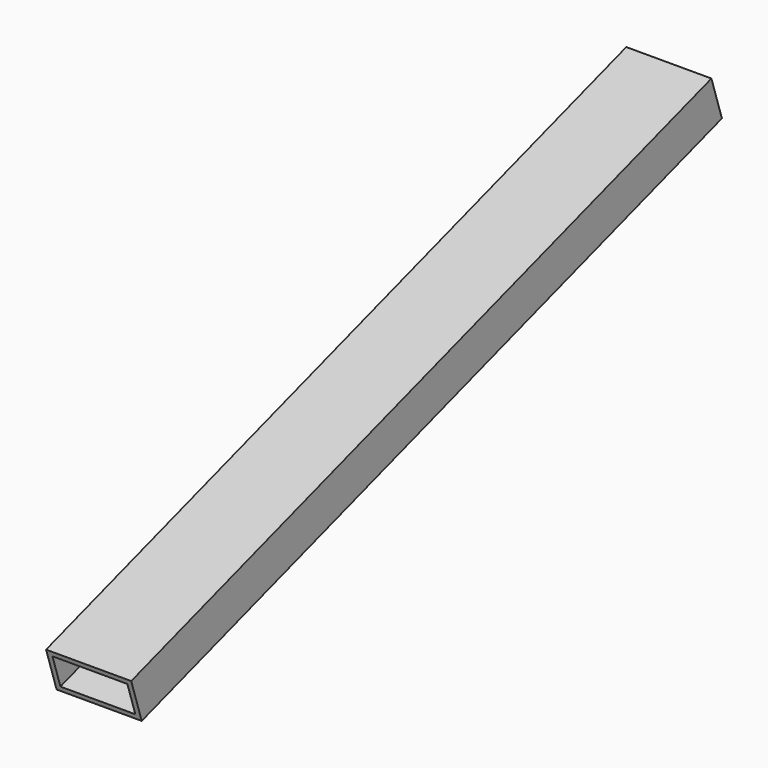
from build123d import *

# Parameters (mm, degrees)
F1_DEPTH = 25
F2_W     = 44
F2_H     = 19
F3_DEPTH = 455.2712231792


# Not quite as in the source:
# - a feature names something its author has since deleted; it is built from what else it names


with BuildPart() as f1:
    # F0 (on Right) → F1 (new body, symmetric)
    with BuildSketch(Plane.YZ):
        Polygon((1862, 545.9546269485), (2050, 607.0395298403), (2042.2745751406, 630.8159427477), (1854.2745751406, 569.7310398559), align=None)
        Polygon((2042.2745751406, 630.8159427477), (2050, 607.0395298403), (2100, 623.2855146519), (2092.2745751406, 647.0619275593), align=None)
        Polygon((2092.2745751406, 647.0619275593), (2100, 623.2855146519), (2288, 684.3704175437), (2280.2745751406, 708.1468304511), align=None)
    extrude(amount=F1_DEPTH, both=True)

    # F2 (on face) → F3 (cut, through all)
    with BuildSketch(Plane(origin=(0, 1844.6468608337, 599.3620976791), x_dir=(1, 0, 0), z_dir=(0, -0.9510565163, -0.3090169944))):
        with Locations((0, -43.6559379653)):
            Rectangle(F2_W, F2_H)
    extrude(amount=-F3_DEPTH, mode=Mode.SUBTRACT)


solid = f1.part
